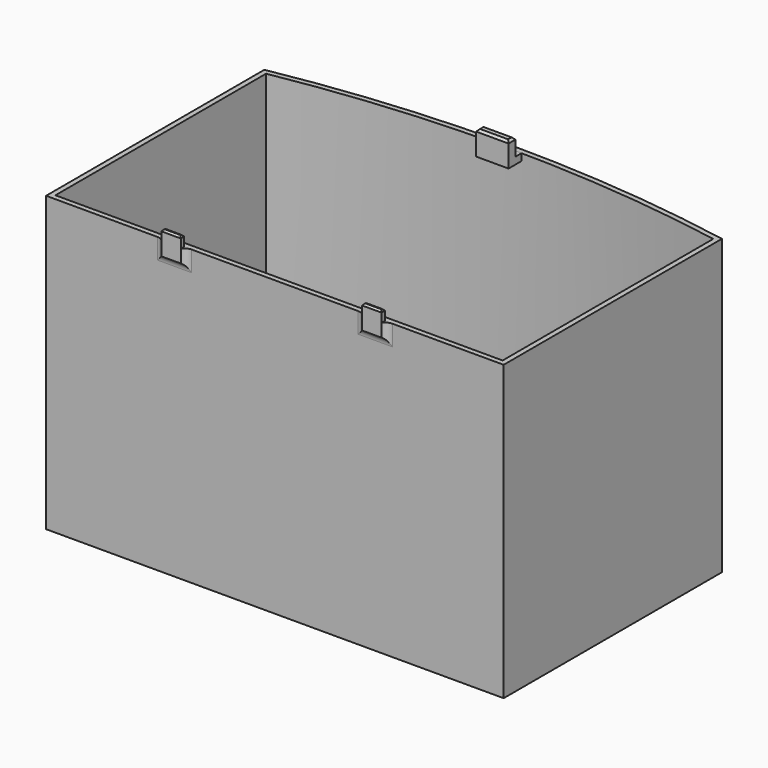
from build123d import *

# Parameters (mm, degrees)
F1_DEPTH     = 68
F2_W         = 4.5
F2_H         = 2.5
F2_H_2       = 3
F3_DEPTH     = 1
F4_T1_DEPTH  = 3
F4_T3_DEPTH  = 4.5
F4_T5_DEPTH  = 4.5
F4_T11_DEPTH = 7.3301270189
F4_T15_DEPTH = 8.8301270189
F4_T22_DEPTH = 8.8301270189
F4_T26_DEPTH = 7.3301270189
F4_T33_DEPTH = 8.8301270189
F4_T37_DEPTH = 7.3301270189
F4_T44_DEPTH = 7.3301270189
F4_T48_DEPTH = 8.8301270189
F5_W         = 7.5
F5_H         = 3.8003136895
F6_DEPTH     = 1.6
F7_W         = 7.5
F7_H         = 2
F8_DEPTH     = 4
F9_SIZE      = 0.5
F10_SIZE     = 0.4


# Not quite as in the source:
# - a fillet or chamfer that OpenCascade refuses, or shapes differently, is made with other operations: its cross-section is extruded or revolved along the edge and cut away or added


with BuildPart() as f1:
    # F0 (on Top) → F1 (new body)
    with BuildSketch(Plane.XY):
        with BuildLine():
            ThreePointArc((61.7473262101, 10.9707194196), (8.7473262101, 15.7712320468), (-44.2526737899, 10.9707194196))
            Line((-44.2526737899, 10.9707194196), (-44.2526737899, -52.2287679532))
            Line((-44.2526737899, -52.2287679532), (61.7473262101, -52.2287679532))
            Line((61.7473262101, -52.2287679532), (61.7473262101, 10.9707194196))
        make_face()
        with BuildLine():
            ThreePointArc((-43.0526737899, 9.9683154894), (8.7473262101, 14.5712320468), (60.5473262101, 9.9683154894))
            Line((60.5473262101, 9.9683154894), (60.5473262101, -51.0287679532))
            Line((60.5473262101, -51.0287679532), (-43.0526737899, -51.0287679532))
            Line((-43.0526737899, -51.0287679532), (-43.0526737899, 9.9683154894))
        make_face(mode=Mode.SUBTRACT)
    extrude(amount=F1_DEPTH)

    # F2 (on face) → F3 (join)
    with BuildSketch(Plane.XZ.offset(52.2287679532)):
        with Locations((-14.5026737899, 69.25)):
            Rectangle(F2_W, F2_H)
        with Locations((31.9973262101, 69.25)):
            Rectangle(F2_W, F2_H)
        with Locations((-14.5026737899, 66.5)):
            Rectangle(F2_W, F2_H_2)
        with Locations((31.9973262101, 66.5)):
            Rectangle(F2_W, F2_H_2)
    extrude(amount=F3_DEPTH)

    # F4: fillet of radius 2 on 6 edges, made by hand

    # F4_s2 → F4_t1 (join)
    with BuildSketch(Plane.XY.offset(65)):
        with BuildLine():
            ThreePointArc((-10.5206229823, -52.2287679532), (-11.5206229823, -52.4967171456), (-12.2526737899, -53.2287679532))
            Line((-12.2526737899, -53.2287679532), (-12.2526737899, -52.2287679532))
            Line((-12.2526737899, -52.2287679532), (-10.5206229823, -52.2287679532))
        make_face()
        with BuildLine():
            ThreePointArc((-18.4847245974, -52.2287679532), (-17.4847245974, -52.4967171456), (-16.7526737899, -53.2287679532))
            Line((-16.7526737899, -53.2287679532), (-16.7526737899, -52.2287679532))
            Line((-16.7526737899, -52.2287679532), (-18.4847245974, -52.2287679532))
        make_face()
        with BuildLine():
            ThreePointArc((28.0152754026, -52.2287679532), (29.0152754026, -52.4967171456), (29.7473262101, -53.2287679532))
            Line((29.7473262101, -53.2287679532), (29.7473262101, -52.2287679532))
            Line((29.7473262101, -52.2287679532), (28.0152754026, -52.2287679532))
        make_face()
        with BuildLine():
            ThreePointArc((35.9793770177, -52.2287679532), (34.9793770177, -52.4967171456), (34.2473262101, -53.2287679532))
            Line((34.2473262101, -53.2287679532), (34.2473262101, -52.2287679532))
            Line((34.2473262101, -52.2287679532), (35.9793770177, -52.2287679532))
        make_face()
    extrude(amount=F4_T1_DEPTH)

    # F4_s4 → F4_t3 (join)
    with BuildSketch(Plane.YZ.offset(-16.7526737899)):
        with BuildLine():
            ThreePointArc((-52.2287679532, 63.2679491924), (-52.4967171456, 64.2679491924), (-53.2287679532, 65))
            Line((-53.2287679532, 65), (-52.2287679532, 65))
            Line((-52.2287679532, 65), (-52.2287679532, 63.2679491924))
        make_face()
    extrude(amount=F4_T3_DEPTH)

    # F4_s6 → F4_t5 (join)
    with BuildSketch(Plane.YZ.offset(29.7473262101)):
        with BuildLine():
            ThreePointArc((-52.2287679532, 63.2679491924), (-52.4967171456, 64.2679491924), (-53.2287679532, 65))
            Line((-53.2287679532, 65), (-52.2287679532, 65))
            Line((-52.2287679532, 65), (-52.2287679532, 63.2679491924))
        make_face()
    extrude(amount=F4_T5_DEPTH)


with BuildPart() as f4_tool9:
    # F4_s10 → F4_t11 (new body)
    with BuildSketch(Plane.XY.offset(60.6698729811)):
        with BuildLine():
            ThreePointArc((-10.5206229823, -52.2287679532), (-11.5206229823, -52.4967171456), (-12.2526737899, -53.2287679532))
            Line((-12.2526737899, -53.2287679532), (-12.2526737899, -52.2287679532))
            Line((-12.2526737899, -52.2287679532), (-10.5206229823, -52.2287679532))
        make_face()
    extrude(amount=F4_T11_DEPTH)

    split(bisect_by=Plane.XY.offset(65), keep=Keep.BOTTOM)


with BuildPart() as f4_tool13:
    # F4_s14 → F4_t15 (new body)
    with BuildSketch(Plane.YZ.offset(-16.7526737899)):
        with BuildLine():
            ThreePointArc((-52.2287679532, 63.2679491924), (-52.4967171456, 64.2679491924), (-53.2287679532, 65))
            Line((-53.2287679532, 65), (-52.2287679532, 65))
            Line((-52.2287679532, 65), (-52.2287679532, 63.2679491924))
        make_face()
    extrude(amount=F4_T15_DEPTH)

    split(bisect_by=Plane.YZ.offset(-12.2526737899), keep=Keep.TOP)


with BuildPart() as f4_tool9_1:
    add(f4_tool9.part)

    # F4_t17: intersect F4_tool13
    add(f4_tool13.part, mode=Mode.INTERSECT)


with BuildPart() as f1_1:
    add(f1.part)

    # F4_t7: union F4_tool9
    add(f4_tool9_1.part)


with BuildPart() as f4_tool20:
    # F4_s21 → F4_t22 (new body)
    with BuildSketch(Plane.YZ.offset(-21.0828008088)):
        with BuildLine():
            ThreePointArc((-52.2287679532, 63.2679491924), (-52.4967171456, 64.2679491924), (-53.2287679532, 65))
            Line((-53.2287679532, 65), (-52.2287679532, 65))
            Line((-52.2287679532, 65), (-52.2287679532, 63.2679491924))
        make_face()
    extrude(amount=F4_T22_DEPTH)

    split(bisect_by=Plane.YZ.offset(-16.7526737899), keep=Keep.BOTTOM)


with BuildPart() as f4_tool24:
    # F4_s25 → F4_t26 (new body)
    with BuildSketch(Plane.XY.offset(68)):
        with BuildLine():
            ThreePointArc((-18.4847245974, -52.2287679532), (-17.4847245974, -52.4967171456), (-16.7526737899, -53.2287679532))
            Line((-16.7526737899, -53.2287679532), (-16.7526737899, -52.2287679532))
            Line((-16.7526737899, -52.2287679532), (-18.4847245974, -52.2287679532))
        make_face()
    extrude(amount=-F4_T26_DEPTH)

    split(bisect_by=Plane.XY.offset(65), keep=Keep.BOTTOM)


with BuildPart() as f4_tool20_1:
    add(f4_tool20.part)

    # F4_t28: intersect F4_tool24
    add(f4_tool24.part, mode=Mode.INTERSECT)


with BuildPart() as f1_2:
    add(f1_1.part)

    # F4_t18: union F4_tool20
    add(f4_tool20_1.part)


with BuildPart() as f4_tool31:
    # F4_s32 → F4_t33 (new body)
    with BuildSketch(Plane.YZ.offset(25.4171991912)):
        with BuildLine():
            ThreePointArc((-52.2287679532, 63.2679491924), (-52.4967171456, 64.2679491924), (-53.2287679532, 65))
            Line((-53.2287679532, 65), (-52.2287679532, 65))
            Line((-52.2287679532, 65), (-52.2287679532, 63.2679491924))
        make_face()
    extrude(amount=F4_T33_DEPTH)

    split(bisect_by=Plane.YZ.offset(29.7473262101), keep=Keep.BOTTOM)


with BuildPart() as f4_tool35:
    # F4_s36 → F4_t37 (new body)
    with BuildSketch(Plane.XY.offset(68)):
        with BuildLine():
            ThreePointArc((28.0152754026, -52.2287679532), (29.0152754026, -52.4967171456), (29.7473262101, -53.2287679532))
            Line((29.7473262101, -53.2287679532), (29.7473262101, -52.2287679532))
            Line((29.7473262101, -52.2287679532), (28.0152754026, -52.2287679532))
        make_face()
    extrude(amount=-F4_T37_DEPTH)

    split(bisect_by=Plane.XY.offset(65), keep=Keep.BOTTOM)


with BuildPart() as f4_tool31_1:
    add(f4_tool31.part)

    # F4_t39: intersect F4_tool35
    add(f4_tool35.part, mode=Mode.INTERSECT)


with BuildPart() as f1_3:
    add(f1_2.part)

    # F4_t29: union F4_tool31
    add(f4_tool31_1.part)


with BuildPart() as f4_tool42:
    # F4_s43 → F4_t44 (new body)
    with BuildSketch(Plane.XY.offset(60.6698729811)):
        with BuildLine():
            ThreePointArc((35.9793770177, -52.2287679532), (34.9793770177, -52.4967171456), (34.2473262101, -53.2287679532))
            Line((34.2473262101, -53.2287679532), (34.2473262101, -52.2287679532))
            Line((34.2473262101, -52.2287679532), (35.9793770177, -52.2287679532))
        make_face()
    extrude(amount=F4_T44_DEPTH)

    split(bisect_by=Plane.XY.offset(65), keep=Keep.BOTTOM)


with BuildPart() as f4_tool46:
    # F4_s47 → F4_t48 (new body)
    with BuildSketch(Plane.YZ.offset(29.7473262101)):
        with BuildLine():
            ThreePointArc((-52.2287679532, 63.2679491924), (-52.4967171456, 64.2679491924), (-53.2287679532, 65))
            Line((-53.2287679532, 65), (-52.2287679532, 65))
            Line((-52.2287679532, 65), (-52.2287679532, 63.2679491924))
        make_face()
    extrude(amount=F4_T48_DEPTH)

    split(bisect_by=Plane.YZ.offset(34.2473262101), keep=Keep.TOP)


with BuildPart() as f4_tool42_1:
    add(f4_tool42.part)

    # F4_t50: intersect F4_tool46
    add(f4_tool46.part, mode=Mode.INTERSECT)


with BuildPart() as f1_4:
    add(f1_3.part)

    # F4_t40: union F4_tool42
    add(f4_tool42_1.part)

    # F10
    f10_edges = [f1_4.edges().sort_by_distance(p)[0] for p in [
        (31.997326, -52.228768, 70.5),
        (29.747326, -52.728768, 70.5),
        (31.997326, -53.228768, 70.5),
        (34.247326, -52.728768, 70.5),
        (-14.502674, -52.228768, 70.5),
        (-16.752674, -52.728768, 70.5),
        (-12.252674, -52.728768, 70.5),
        (-14.502674, -53.228768, 70.5),
    ]]
    chamfer(f10_edges, length=F10_SIZE)


with BuildPart() as f6:
    # F5 (on face) → F6 (new body)
    with BuildSketch(Plane.XY.offset(68)):
        with Locations((8.7473262101, 12.6471399452)):
            Rectangle(F5_W, F5_H)
    extrude(amount=-F6_DEPTH)

    # F7 (on face) → F8 (join)
    with BuildSketch(Plane.XY.offset(68)):
        with Locations((8.7473262101, 11.7469831005)):
            Rectangle(F7_W, F7_H)
    extrude(amount=F8_DEPTH)

    # F9
    f9_edges = [f6.edges().sort_by_distance(p)[0] for p in [
        (4.997326, 11.746983, 72),
        (8.747326, 10.746983, 72),
        (8.747326, 12.746983, 72),
        (12.497326, 11.746983, 72),
    ]]
    chamfer(f9_edges, length=F9_SIZE)


solid = Compound([f1_4.part, f6.part])
